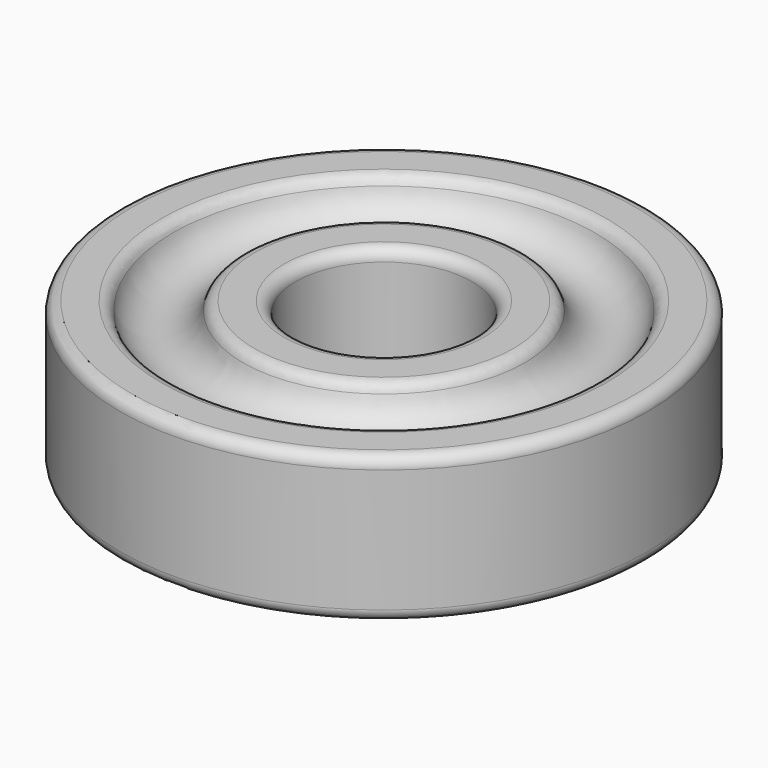
from build123d import *

# Parameters (mm, degrees)
F2_R = 0.2


with BuildPart() as f1:
    # F0 (on Front) → F1 (revolve)
    with BuildSketch(Plane.XZ):
        with BuildLine():
            Line((-95.475864, 27.369046), (-95.475864, 24.869046))
            Line((-95.475864, 24.869046), (-94.5922780685, 24.869046))
            ThreePointArc((-94.5922780685, 24.869046), (-93.975864, 25.4854600685), (-93.3594499315, 24.869046))
            Line((-93.3594499315, 24.869046), (-92.475864, 24.869046))
            Line((-92.475864, 24.869046), (-92.475864, 27.369046))
            Line((-92.475864, 27.369046), (-93.3594499315, 27.369046))
            ThreePointArc((-93.3594499315, 27.369046), (-93.975864, 26.7526319315), (-94.5922780685, 27.369046))
            Line((-94.5922780685, 27.369046), (-95.475864, 27.369046))
        make_face()
    revolve(axis=Axis((-90.975864, 0, 26.1190455), (0, 0, 1)))

    # F2
    f2_edges = [f1.edges().sort_by_distance(p)[0] for p in [
        (-86.475864, 0, 27.369046),
        (-86.475864, 0, 24.869046),
        (-95.475864, 0, 26.119046),
        (-89.475864, 0, 24.869046),
        (-88.592278, 0, 27.369046),
        (-88.592278, 0, 24.869046),
        (-87.35945, 0, 27.369046),
        (-89.475864, 0, 27.369046),
    ]]
    fillet(f2_edges, radius=F2_R)


solid = f1.part
